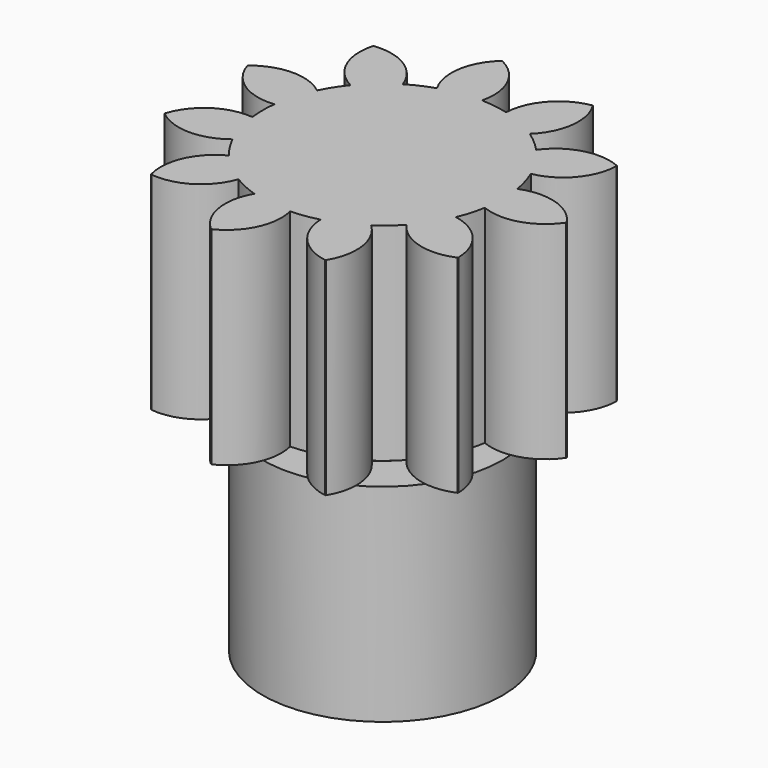
from build123d import *

# Parameters (mm, degrees)
F0_R      = 14.732
F1_DEPTH  = 25.4
F3_DEPTH  = 25.4
F4_COUNT  = 11
F6_DEPTH  = 12.7
F8_DEPTH  = 12.7
F9_R      = 9.398
F10_DEPTH = 2.794
F11_R     = 14.732
F12_DEPTH = 25.4


with BuildPart() as f1:
    # F0 (on Top) → F1 (new body)
    with BuildSketch(Plane.XY):
        Circle(F0_R)
    extrude(amount=F1_DEPTH)

    # F2 (on face) → F3 (join, through all)
    with BuildSketch(Plane.XY.offset(25.4)):
        with BuildLine():
            Line((-4.5369443263, 13.978875159), (0.3913960902, 14.6914813287))
            ThreePointArc((0.3913960902, 14.6914813287), (-0.0382185694, 19.133161975), (-3.1729441601, 22.3091013936))
            Line((-3.1729441601, 22.3091013936), (-3.2763966599, 22.2941428308))
            ThreePointArc((-3.2763966599, 22.2941428308), (-5.3830975977, 18.3603270143), (-4.5369443263, 13.978875159))
        make_face()
    extrude(amount=-F3_DEPTH)

    # F4: F1 ×11 about axis
    f4_axis = Axis((0, 0, 25.4), (0, 0, -1))


with BuildPart() as f1_1:
    add(f1.part)
    for i in range(1, F4_COUNT):
        add(f1.part.rotate(f4_axis, i * 360 / F4_COUNT))

    # F5 (on face) → F6 (cut)
    with BuildSketch(Plane(origin=(0, 0, 0), x_dir=(1, 0, 0), z_dir=(0, 0, -1))):
        with BuildLine():
            Line((1.905, -8.597513929), (1.905, -6.057513929))
            ThreePointArc((1.905, -6.057513929), (0, 6.35), (-1.905, -6.057513929))
            Line((-1.905, -6.057513929), (-1.905, -8.597513929))
            Line((-1.905, -8.597513929), (1.905, -8.597513929))
        make_face()
    extrude(amount=-F6_DEPTH, mode=Mode.SUBTRACT)


with BuildPart() as f8:
    # F7 (on face) → F8 (new body, through all)
    with BuildSketch(Plane(origin=(0, 0, 12.7), x_dir=(1, 0, 0), z_dir=(0, 0, -1))):
        with BuildLine():
            Line((1.524, -8.3020531043), (1.524, -5.5080531043))
            ThreePointArc((1.524, -5.5080531043), (0, 5.715), (-1.524, -5.5080531043))
            Line((-1.524, -5.5080531043), (-1.524, -8.3020531043))
            Line((-1.524, -8.3020531043), (1.524, -8.3020531043))
        make_face()
    extrude(amount=F8_DEPTH)

    # F9 (on face) → F10 (join)
    with BuildSketch(Plane(origin=(0, 0, 0), x_dir=(1, 0, 0), z_dir=(0, 0, -1))):
        Circle(F9_R)
    extrude(amount=F10_DEPTH)

    # F11 (on face) → F12 (join)
    with BuildSketch(Plane(origin=(0, 0, -2.794), x_dir=(1, 0, 0), z_dir=(0, 0, -1))):
        Circle(F11_R)
    extrude(amount=F12_DEPTH)


solid = Compound([f1_1.part, f8.part])
